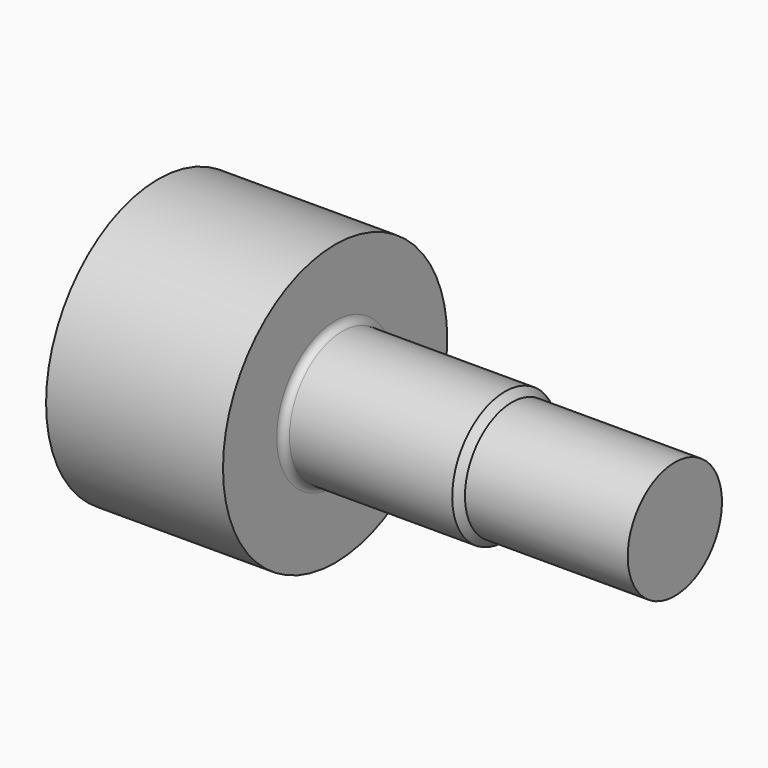
from build123d import *

# Parameters (mm, degrees)
F0_W     = 2.921
F0_H     = 1.05664
F2_R     = 0.127
F3_SIZE2 = 0.12699
F3_SIZE  = 0.12699


# Not quite as in the source:
# - a fillet or chamfer is up to 0.001 mm smaller than in the source, because OpenCascade refuses the exact size


with BuildPart() as f1:
    # F0 (on Front) → F1 (revolve)
    with BuildSketch(Plane.XZ):
        Polygon((-3.175, 0), (0, 0), (0, 1.18364), (0, 2.5146), (-3.175, 2.5146), align=None)
        Polygon((0, 1.18364), (0, 0), (3.175, 0), (3.175, 1.05664), (3.175, 1.18364), align=None)
        with Locations((4.6355, 0.52832)):
            Rectangle(F0_W, F0_H)
    revolve(axis=Axis((-1.5875, 0, 0), (-1, 0, 0)))

    # F2
    f2_edges = [f1.edges().sort_by_distance(p)[0] for p in [
        (0, 0, -1.18364),
    ]]
    fillet(f2_edges, radius=F2_R)

    # F3 (size 0.127 and 0.127 in the source; OpenCascade refuses exactly that, so slightly less here)
    f3_edges = [f1.edges().sort_by_distance(p)[0] for p in [
        (3.175, 0, -1.18364),
    ]]
    chamfer(f3_edges, length=F3_SIZE, length2=F3_SIZE2)


solid = f1.part
